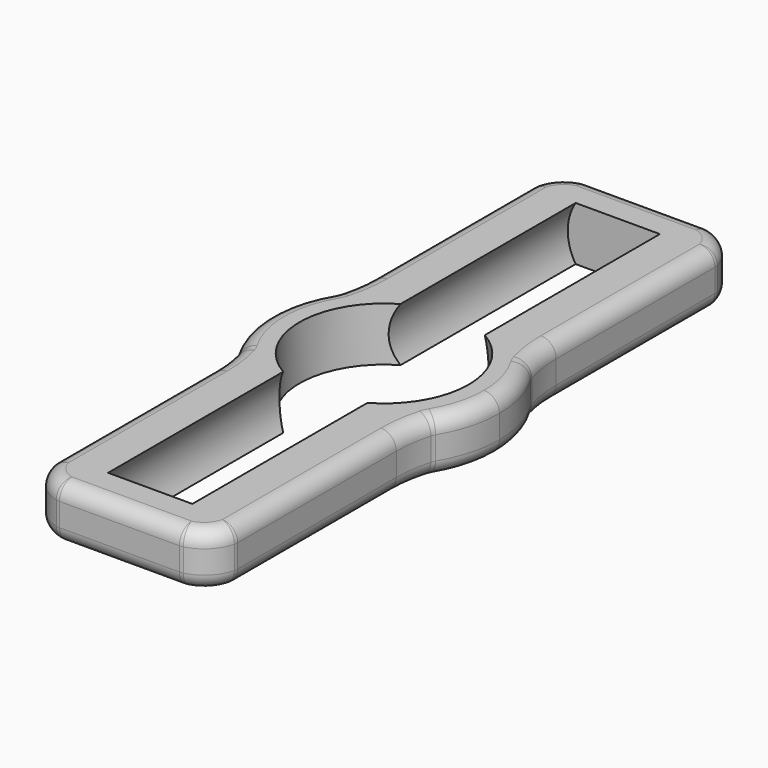
from build123d import *

# Parameters (mm, degrees)
F1_DEPTH = 3.5
F2_R     = 6.5
F3_DEPTH = 38
F4_F1_R  = 2
F4_F2_R  = 2
F4_F3_R  = 2
F4_F4_R  = 2
F4_F5_R  = 2
F4_F6_R  = 2
F4_F7_R  = 2
F4_F8_R  = 2
F4_F9_R  = 2
F4_F10_R = 2
F4_F11_R = 2
F4_F12_R = 2
F4_F13_R = 2
F4_F14_R = 2


with BuildPart() as f1:
    # F0 (on Top) → F1 (new body, symmetric)
    with BuildSketch(Plane.XY):
        with BuildLine():
            ThreePointArc((-12.7367740715, 7.9230414774), (-8.9834574186, 12.0123891382), (-4, 14.4568322948))
            Line((-4, 14.4568322948), (-4, 43))
            Line((-4, 43), (-8, 43))
            ThreePointArc((-8, 43), (-10.6199177052, 41.6199177052), (-12, 39))
            Line((-12, 39), (-12, 13))
            ThreePointArc((-12, 13), (-12.1851532241, 10.4349296368), (-12.7367740715, 7.9230414774))
        make_face()
        with BuildLine():
            Line((4, 43), (4, 14.4568322948))
            ThreePointArc((4, 14.4568322948), (8.9834574186, 12.0123891382), (12.7367740715, 7.9230414774))
            ThreePointArc((12.7367740715, 7.9230414774), (12.1851532241, 10.4349296368), (12, 13))
            Line((12, 13), (12, 39))
            ThreePointArc((12, 39), (10.6199177052, 41.6199177052), (8, 43))
            Line((8, 43), (4, 43))
        make_face()
        with BuildLine():
            ThreePointArc((-4, 14.4568322948), (-2.0183552187, 14.8635877974), (0, 15))
            ThreePointArc((0, 15), (2.0183552187, 14.8635877974), (4, 14.4568322948))
            Line((4, 14.4568322948), (4, 43))
            Line((4, 43), (-4, 43))
            Line((-4, 43), (-4, 14.4568322948))
        make_face()
        with BuildLine():
            ThreePointArc((4, 14.4568322948), (2.0183552187, 14.8635877974), (0, 15))
            ThreePointArc((0, 15), (-2.0183552187, 14.8635877974), (-4, 14.4568322948))
            ThreePointArc((-4, 14.4568322948), (-8.9834574186, 12.0123891382), (-12.7367740715, 7.9230414774))
            ThreePointArc((-12.7367740715, 7.9230414774), (-15, 0), (-12.7367740715, -7.9230414774))
            ThreePointArc((-12.7367740715, -7.9230414774), (-8.9834574186, -12.0123891382), (-4, -14.4568322948))
            ThreePointArc((-4, -14.4568322948), (0, -15), (4, -14.4568322948))
            ThreePointArc((4, -14.4568322948), (8.9834574186, -12.0123891382), (12.7367740715, -7.9230414774))
            ThreePointArc((12.7367740715, -7.9230414774), (14.4230997201, -4.1199750562), (15, 0))
            ThreePointArc((15, 0), (14.4230997201, 4.1199750562), (12.7367740715, 7.9230414774))
            ThreePointArc((12.7367740715, 7.9230414774), (8.9834574186, 12.0123891382), (4, 14.4568322948))
        make_face()
        with BuildLine():
            ThreePointArc((0, 11), (7.7781745931, 7.7781745931), (11, 0))
            ThreePointArc((11, 0), (-7.7781745931, -7.7781745931), (0, 11))
        make_face(mode=Mode.SUBTRACT)
        with BuildLine():
            ThreePointArc((12, -13), (12.1851532241, -10.4349296368), (12.7367740715, -7.9230414774))
            ThreePointArc((12.7367740715, -7.9230414774), (8.9834574186, -12.0123891382), (4, -14.4568322948))
            Line((4, -14.4568322948), (4, -43))
            Line((4, -43), (8, -43))
            ThreePointArc((8, -43), (10.6199177052, -41.6199177052), (12, -39))
            Line((12, -39), (12, -13))
        make_face()
        with BuildLine():
            ThreePointArc((4, -14.4568322948), (0, -15), (-4, -14.4568322948))
            Line((-4, -14.4568322948), (-4, -43))
            Line((-4, -43), (4, -43))
            Line((4, -43), (4, -14.4568322948))
        make_face()
        with BuildLine():
            ThreePointArc((-4, -14.4568322948), (-8.9834574186, -12.0123891382), (-12.7367740715, -7.9230414774))
            ThreePointArc((-12.7367740715, -7.9230414774), (-12.1851532241, -10.4349296368), (-12, -13))
            Line((-12, -13), (-12, -39))
            ThreePointArc((-12, -39), (-10.6199177052, -41.6199177052), (-8, -43))
            Line((-8, -43), (-4, -43))
            Line((-4, -43), (-4, -14.4568322948))
        make_face()
    extrude(amount=F1_DEPTH, both=True)

    # F2 (on Front) → F3 (cut, symmetric)
    with BuildSketch(Plane.XZ):
        Circle(F2_R)
    extrude(amount=F3_DEPTH, both=True, mode=Mode.SUBTRACT)

    # F4: fillet of radius 2 on 48 edges, made by hand

    # F4_f1
    f4_f1_edges = [f1.edges().sort_by_distance(p)[0] for p in [
        (12.7367740715, 7.9230414774, 0),
    ]]
    fillet(f4_f1_edges, radius=F4_F1_R)

    # F4_f2
    f4_f2_edges = [f1.edges().sort_by_distance(p)[0] for p in [
        (12.7367740715, -7.9230414774, 0),
    ]]
    fillet(f4_f2_edges, radius=F4_F2_R)

    # F4_f3
    f4_f3_edges = [f1.edges().sort_by_distance(p)[0] for p in [
        (12, -39, 0),
    ]]
    fillet(f4_f3_edges, radius=F4_F3_R)

    # F4_f4
    f4_f4_edges = [f1.edges().sort_by_distance(p)[0] for p in [
        (8, -43, 0),
    ]]
    fillet(f4_f4_edges, radius=F4_F4_R)

    # F4_f5
    f4_f5_edges = [f1.edges().sort_by_distance(p)[0] for p in [
        (-8, -43, 0),
    ]]
    fillet(f4_f5_edges, radius=F4_F5_R)

    # F4_f6
    f4_f6_edges = [f1.edges().sort_by_distance(p)[0] for p in [
        (-12, -39, 0),
    ]]
    fillet(f4_f6_edges, radius=F4_F6_R)

    # F4_f7
    f4_f7_edges = [f1.edges().sort_by_distance(p)[0] for p in [
        (-12.7367740715, -7.9230414774, 0),
    ]]
    fillet(f4_f7_edges, radius=F4_F7_R)

    # F4_f8
    f4_f8_edges = [f1.edges().sort_by_distance(p)[0] for p in [
        (-12.7367740715, 7.9230414774, 0),
    ]]
    fillet(f4_f8_edges, radius=F4_F8_R)

    # F4_f9
    f4_f9_edges = [f1.edges().sort_by_distance(p)[0] for p in [
        (-12, 39, 0),
    ]]
    fillet(f4_f9_edges, radius=F4_F9_R)

    # F4_f10
    f4_f10_edges = [f1.edges().sort_by_distance(p)[0] for p in [
        (-8, 43, 0),
    ]]
    fillet(f4_f10_edges, radius=F4_F10_R)

    # F4_f11
    f4_f11_edges = [f1.edges().sort_by_distance(p)[0] for p in [
        (8, 43, 0),
    ]]
    fillet(f4_f11_edges, radius=F4_F11_R)

    # F4_f12
    f4_f12_edges = [f1.edges().sort_by_distance(p)[0] for p in [
        (12, 39, 0),
    ]]
    fillet(f4_f12_edges, radius=F4_F12_R)

    # F4_f13
    f4_f13_edges = [f1.edges().sort_by_distance(p)[0] for p in [
        (0, -43, -3.5),
    ]]
    fillet(f4_f13_edges, radius=F4_F13_R)

    # F4_f14
    f4_f14_edges = [f1.edges().sort_by_distance(p)[0] for p in [
        (0, -43, 3.5),
    ]]
    fillet(f4_f14_edges, radius=F4_F14_R)


solid = f1.part
